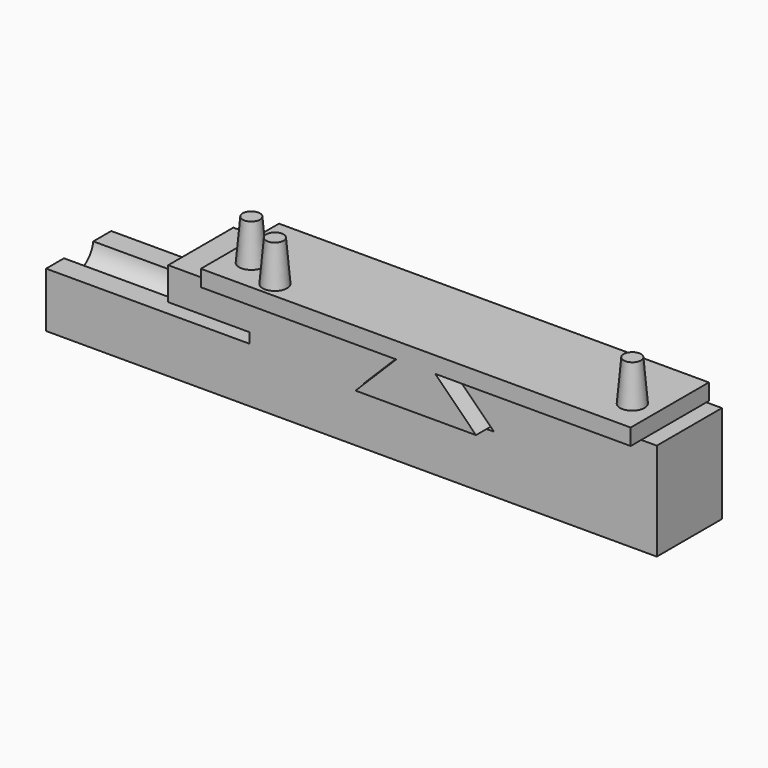
from build123d import *

# Parameters (mm, degrees)
F1_DEPTH    = 10
F2_W        = 25
F2_H        = 4.5
F3_DEPTH    = 2.5
F6_DEPTH    = 10.001
F7_T1_DEPTH = 32.3950997289
F9_DEPTH    = 12
F10_R       = 1.5
F11_DEPTH   = 5
F11_TAPER   = 5


# Not quite as in the source:
# - a fillet or chamfer that OpenCascade refuses, or shapes differently, is made with other operations: its cross-section is extruded or revolved along the edge and cut away or added


with BuildPart() as f1:
    # F0 (on Front) → F1 (new body)
    with BuildSketch(Plane.XZ):
        Polygon((0, -12), (0, 0), (-60, 0), (-60, -4), (-50, -4), (-50, -5.25), (-75, -5.25), (-75, -12), (-70, -12), (-5, -12), align=None)
    extrude(amount=F1_DEPTH)

    # F2 (on face) → F3 (cut)
    with BuildSketch(Plane.XY.offset(-5.25)):
        with Locations((-62.5, -5)):
            Rectangle(F2_W, F2_H)
    extrude(amount=-F3_DEPTH, mode=Mode.SUBTRACT)

    # F5 (on face) → F6 (cut, through all)
    with BuildSketch(Plane.XZ.offset(10)):
        Polygon((-28, 0), (-31, 0), (-36, -5), (-28, -5), (-20, -5), (-25, 0), align=None)
    extrude(amount=-F6_DEPTH, mode=Mode.SUBTRACT)

    # F7: fillet of radius 3 on 2 edges, made by hand

    # F7_s2 → F7_t1 (join)
    with BuildSketch(Plane.YZ.offset(-75)):
        with BuildLine():
            ThreePointArc((-5.7080398916, -7.75), (-3.7715482184, -7.0412878475), (-2.75, -5.25))
            Line((-2.75, -5.25), (-2.75, -7.75))
            Line((-2.75, -7.75), (-5.7080398916, -7.75))
        make_face()
        with BuildLine():
            ThreePointArc((-7.25, -5.25), (-6.2284517816, -7.0412878475), (-4.2919601084, -7.75))
            Line((-4.2919601084, -7.75), (-7.25, -7.75))
            Line((-7.25, -7.75), (-7.25, -5.25))
        make_face()
    extrude(amount=F7_T1_DEPTH)


with BuildPart() as f9:
    # F8 (on Front) → F9 (new body)
    with BuildSketch(Plane.XZ):
        Polygon((-20.6035533906, -4.75), (-25.6035533906, 0.25), (-1.6035533906, 0.25), (-1.6035533906, 2.25), (-54.3964466094, 2.25), (-54.3964466094, 0.25), (-30.3964466094, 0.25), (-35.3964466094, -4.75), align=None)
    extrude(amount=F9_DEPTH)


with BuildPart() as f11:
    # F10 (on face) → F11 (new body)
    with BuildSketch(Plane.XY.offset(2.25)):
        with Locations((-46.8964466094, -10)):
            Circle(F10_R)
    extrude(amount=F11_DEPTH, taper=F11_TAPER)


with BuildPart() as f11b:
    # F10 (on face) → F11, piece 2 (new body)
    with BuildSketch(Plane.XY.offset(2.25)):
        with Locations((-51.3964466094, -8)):
            Circle(F10_R)
    extrude(amount=F11_DEPTH, taper=F11_TAPER)


with BuildPart() as f11c:
    # F10 (on face) → F11, piece 3 (new body)
    with BuildSketch(Plane.XY.offset(2.25)):
        with Locations((-4.6035533906, -8)):
            Circle(F10_R)
    extrude(amount=F11_DEPTH, taper=F11_TAPER)


solid = Compound([f1.part, f9.part, f11.part, f11b.part, f11c.part])
